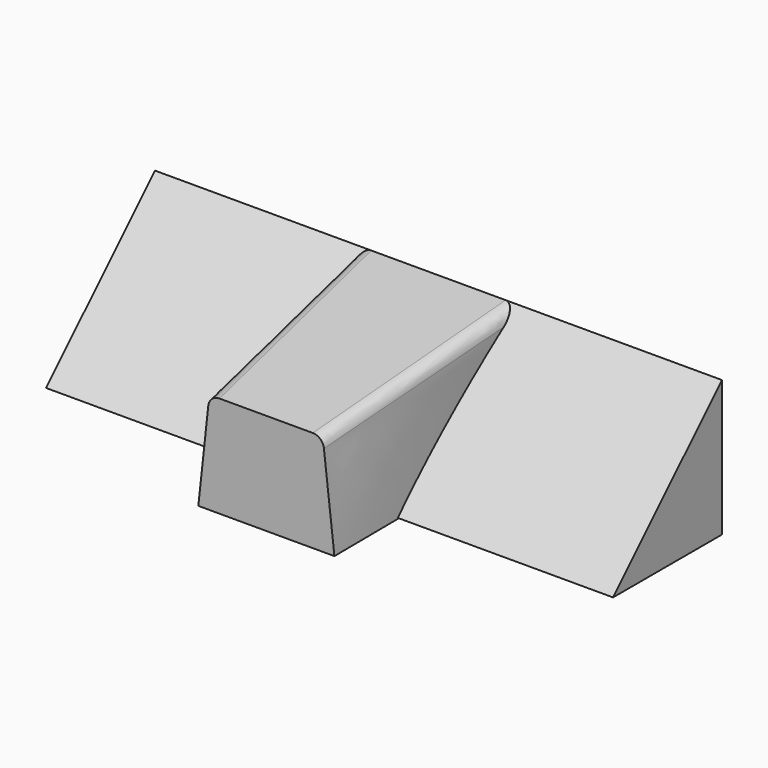
from build123d import *

# Parameters (mm, degrees)
F0_W     = 250
F0_H     = 60
F1_DEPTH = 60
F3_DEPTH = 250
F8_R     = 5


with BuildPart() as f1:
    # F0 (on Front) → F1 (new body)
    with BuildSketch(Plane.XZ):
        Rectangle(F0_W, F0_H)
    extrude(amount=F1_DEPTH)

    # F2 (on face) → F3 (cut)
    with BuildSketch(Plane.YZ.offset(125)):
        Polygon((-60, -30), (0, 30), (-60, 30), align=None)
    extrude(amount=-F3_DEPTH, mode=Mode.SUBTRACT)

    # F4 (on face) → F7 section 0
    with BuildSketch(Plane(origin=(0, 0, 0), x_dir=(-1, 0, 0), z_dir=(0, 1, 0))):
        Polygon((35, 30), (-35, 30), (-30, -30), (30, -30), align=None)
    # F6 (on offset) → F7 section 1
    with BuildSketch(Plane.XZ.offset(95)):
        Polygon((25, 14.1158560291), (-25, 14.1158560291), (-29.863614589, -30.5979736149), (30.136385411, -30.5979736149), align=None)
    loft()

    # F8
    f8_edges = [f1.edges().sort_by_distance(p)[0] for p in [
        (30, -47.5, 22.057928),
        (-30, -47.5, 22.057928),
    ]]
    fillet(f8_edges, radius=F8_R)


solid = f1.part
